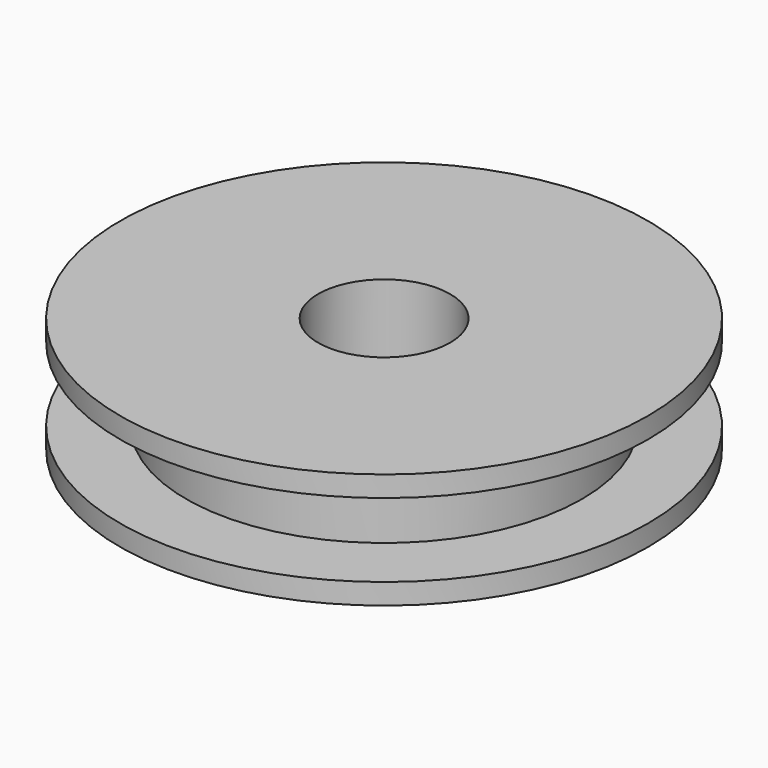
from build123d import *

# Parameters (mm, degrees)
F0_R     = 12.7
F0_R_2   = 3.175
F1_DEPTH = 1.00000054
F2_R     = 9.525
F2_R_2   = 3.175
F3_DEPTH = 3.556
F4_R     = 12.7
F4_R_2   = 9.525
F4_R_3   = 3.175
F5_DEPTH = 1.00000054


# Not quite as in the source:
# - a feature names something its author has since deleted; it is built from what else it names


with BuildPart() as f1:
    # F0 (on Top) → F1 (new body)
    with BuildSketch(Plane.XY):
        Circle(F0_R)
        Circle(F0_R_2, mode=Mode.SUBTRACT)
    extrude(amount=F1_DEPTH)

    # F2 (on face) → F3 (join)
    with BuildSketch(Plane.XY.offset(1.00000054)):
        Circle(F2_R)
        Circle(F2_R_2, mode=Mode.SUBTRACT)
    extrude(amount=F3_DEPTH)

    # F4 (on face) → F5 (join)
    with BuildSketch(Plane.XY.offset(4.55600054)):
        Circle(F4_R)
        Circle(F4_R_2, mode=Mode.SUBTRACT)
        Circle(F4_R_2)
        Circle(F4_R_3, mode=Mode.SUBTRACT)
    extrude(amount=F5_DEPTH)


solid = f1.part
